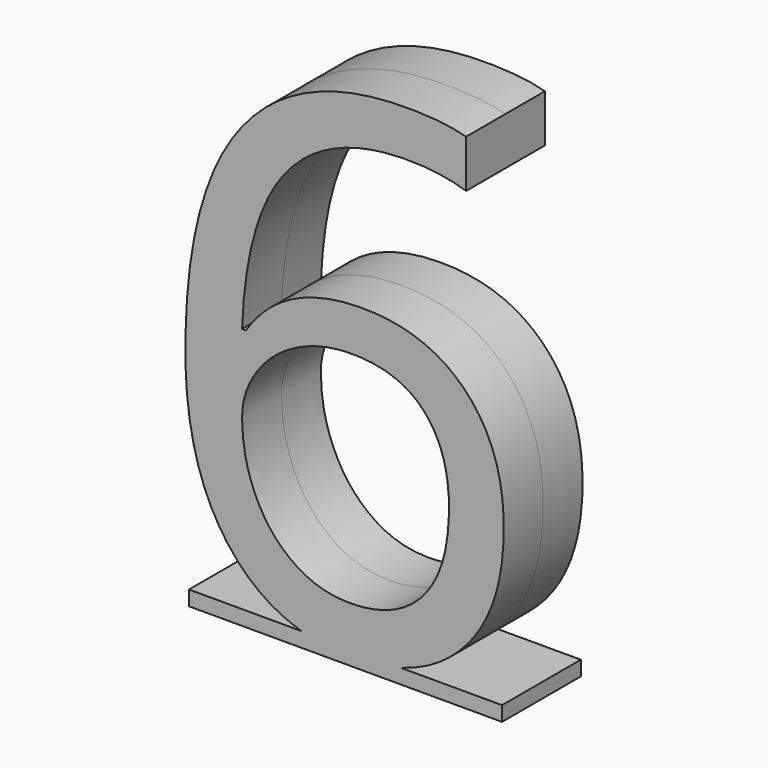
from build123d import *

# Parameters (mm, degrees)
F0_TEXT_SIZE  = 138.8888888889
F1_DEPTH      = 10
F1_DEPTH_BACK = 10
F2_W          = 63.5907118056
F2_H          = 20
F3_DEPTH      = 3


# Not quite as in the source:
# - Text() gives the source's letters only with a copy of the font that has no kerning and outlines rounded to 1/6400 em; it was checked with that copy


with BuildPart() as f1:
    # F0 (on Front) → F1 (new body, two sides)
    with BuildSketch(Plane.XZ) as f1_sk:
        with Locations((-40.8203125, 0)):
            Text('6', F0_TEXT_SIZE, font='Open Sans', text_align=(TextAlign.LEFT, TextAlign.BOTTOM))
    extrude(amount=F1_DEPTH)
    extrude(f1_sk.sketch, amount=-F1_DEPTH_BACK)

    # F2 (on Top) → F3 (join)
    with BuildSketch(Plane.XY):
        with Locations((-0.3465711806, 0)):
            Rectangle(F2_W, F2_H)
    extrude(amount=-F3_DEPTH)


solid = f1.part
